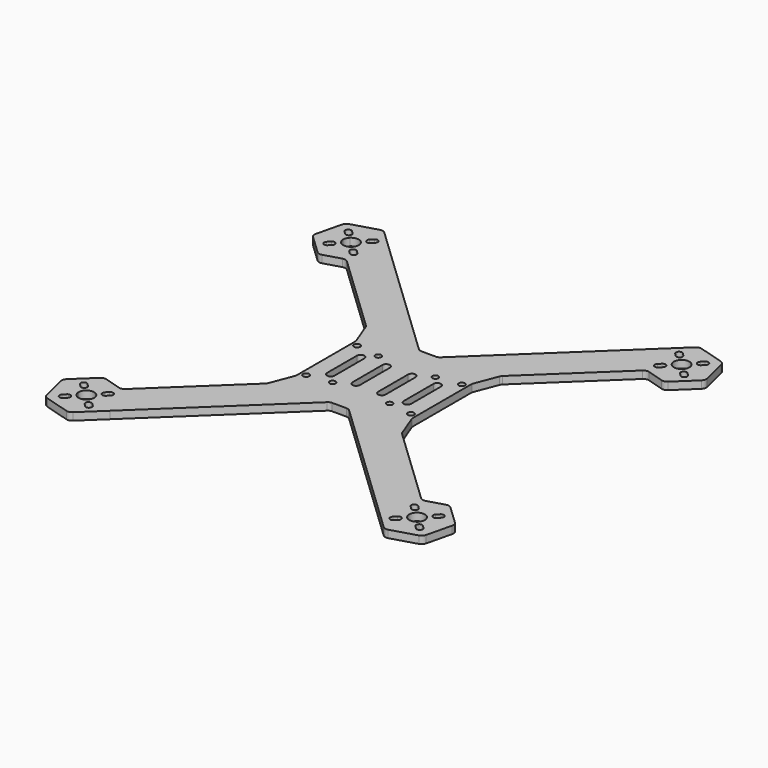
from build123d import *

# Parameters (mm, degrees)
F0_R     = 1.6
F0_R_2   = 1.65
F1_DEPTH = 4
F2_R     = 3


# Not quite as in the source:
# - a feature names something its author has since deleted; it is built from what else it names


with BuildPart() as f1:
    # F0 (on Top) → F1 (new body)
    with BuildSketch(Plane.XY):
        with BuildLine():
            Line((18.4368398041, 0), (18.4368398041, 10))
            ThreePointArc((18.4368398041, 10), (20.4368398041, 12), (22.4368398041, 10))
            Line((22.4368398041, 10), (22.4368398041, 0))
            Line((22.4368398041, 0), (31, 0))
            Line((31, 0), (31, 17))
            Line((31, 17), (31, 20))
            Line((31, 20), (36.0206841705, 33.0998521633))
            Line((36.0206841705, 33.0998521633), (80.2630744621, 75.1477559326))
            Line((80.2630744621, 75.1477559326), (75.833487988, 76.4562271784))
            Line((75.833487988, 76.4562271784), (71.7773983702, 93.2951148202))
            Line((71.7773983702, 93.2951148202), (5, 29.8299719532))
            Line((5, 29.8299719532), (0, 29.8299719532))
            Line((0, 29.8299719532), (0, 0))
            Line((0, 0), (4.865056935, 0))
            Line((4.865056935, 0), (4.865056935, 10))
            ThreePointArc((4.865056935, 10), (6.865056935, 12), (8.865056935, 10))
            Line((8.865056935, 10), (8.865056935, 0))
            Line((8.865056935, 0), (18.4368398041, 0))
        make_face()
        with Locations((15.25, 15.25)):
            Circle(F0_R, mode=Mode.SUBTRACT)
        with Locations((28, 17)):
            Circle(F0_R_2, mode=Mode.SUBTRACT)
        Polygon((84.3322580305, 105.2272352901), (71.7773983702, 93.2951148202), (75.833487988, 76.4562271784), (80.2630744621, 75.1477559326), (92.4444372661, 71.5494600065), (104.9992969265, 83.4815804764), (100.9432073087, 100.3204681182), align=None)
        with BuildLine():
            ThreePointArc((82.4486506864, 80.1859089866), (80.1859089866, 80.1859089866), (80.1859089866, 82.4486506864))
            Line((80.1859089866, 82.4486506864), (81.6001225489, 83.8628642487))
            ThreePointArc((81.6001225489, 83.8628642487), (83.8628642487, 83.8628642487), (83.8628642487, 81.6001225489))
            Line((83.8628642487, 81.6001225489), (82.4486506864, 80.1859089866))
        make_face(mode=Mode.SUBTRACT)
        with BuildLine():
            ThreePointArc((91.3228407902, 91.3228407902), (92.2224477082, 89.9764838926), (92.5383476483, 88.3883476483))
            ThreePointArc((92.5383476483, 88.3883476483), (84.5542475884, 86.800211404), (91.3228407902, 91.3228407902))
        make_face(mode=Mode.SUBTRACT)
        with BuildLine():
            Line((94.3280446103, 80.1859089866), (92.9138310479, 81.6001225489))
            ThreePointArc((92.9138310479, 81.6001225489), (92.9138310479, 83.8628642487), (95.1765727477, 83.8628642487))
            Line((95.1765727477, 83.8628642487), (96.5907863101, 82.4486506864))
            ThreePointArc((96.5907863101, 82.4486506864), (96.5907863101, 80.1859089866), (94.3280446103, 80.1859089866))
        make_face(mode=Mode.SUBTRACT)
        with BuildLine():
            Line((81.6001225489, 92.9138310479), (80.1859089866, 94.3280446103))
            ThreePointArc((80.1859089866, 94.3280446103), (80.1859089866, 96.5907863101), (82.4486506864, 96.5907863101))
            Line((82.4486506864, 96.5907863101), (83.8628642487, 95.1765727477))
            ThreePointArc((83.8628642487, 95.1765727477), (83.8628642487, 92.9138310479), (81.6001225489, 92.9138310479))
        make_face(mode=Mode.SUBTRACT)
        with BuildLine():
            ThreePointArc((95.1765727477, 92.9138310479), (94.0452018978, 92.4452018978), (92.9138310479, 92.9138310479))
            ThreePointArc((92.9138310479, 92.9138310479), (92.4452018978, 94.0452018978), (92.9138310479, 95.1765727477))
            Line((92.9138310479, 95.1765727477), (94.3280446103, 96.5907863101))
            ThreePointArc((94.3280446103, 96.5907863101), (96.5907863101, 96.5907863101), (96.5907863101, 94.3280446103))
            Line((96.5907863101, 94.3280446103), (95.1765727477, 92.9138310479))
        make_face(mode=Mode.SUBTRACT)
    extrude(amount=F1_DEPTH)

    # F2
    f2_edges = [f1.edges().sort_by_distance(p)[0] for p in [
        (18.43684, 10, 2),
        (80.263074, 75.147756, 2),
        (92.444437, 71.54946, 2),
        (104.999297, 83.48158, 2),
        (100.943207, 100.320468, 2),
        (84.332258, 105.227235, 2),
        (5, 29.829972, 2),
        (36.020684, 33.099852, 2),
    ]]
    fillet(f2_edges, radius=F2_R)

    # F3: F1 across plane


with BuildPart() as f1_1:
    add(f1.part)
    add(f1.part.mirror(Plane.YZ))

    # F4: F1 across plane


with BuildPart() as f1_2:
    add(f1_1.part)
    add(f1_1.part.mirror(Plane.XZ))


solid = f1_2.part
